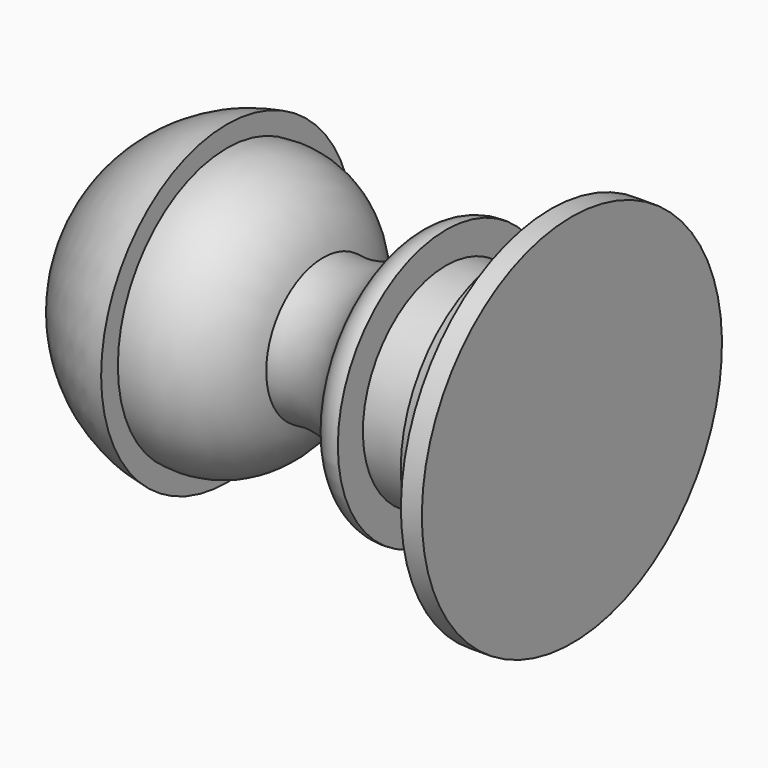
from build123d import *

# Parameters (mm, degrees)
F2_SCALE = 1.7


# Not quite as in the source:
# - a feature names something its author has since deleted; it is built from what else it names


with BuildPart() as f1:
    # F0 (on Front) → F1 (revolve)
    with BuildSketch(Plane.XZ):
        with BuildLine():
            Line((-7.3886374691, 0.0288757618), (0, 0.0425738979))
            Line((0, 0.0425738979), (0, 9))
            Line((0, 9), (-1, 9))
            ThreePointArc((-1, 9), (-1.5826778103, 7.4161422482), (-3, 6.5))
            Line((-3, 6.5), (-3, 5))
            Line((-3, 5), (-6, 5))
            Line((-6, 5), (-6, 6.5))
            ThreePointArc((-6, 6.5), (-6.9250133416, 6.2625200124), (-7.5, 5.5))
            Line((-7.5, 5.5), (-7.5, 0.0286693017))
            Line((-7.5, 0.0286693017), (-7.3886374691, 0.0288757618))
        make_face()
        with BuildLine():
            Line((-15.3639473664, 0.0140899666), (-7.5, 0.0286693017))
            Line((-7.5, 0.0286693017), (-7.5, 5.5))
            ThreePointArc((-7.5, 5.5), (-9.3734949345, 3.8129508491), (-11.8646939118, 3.4255934394))
            ThreePointArc((-11.8646939118, 3.4255934394), (-13.5762184414, 5.8486067414), (-16.4624222987, 6.534272091))
            Line((-16.4624222987, 6.534272091), (-16.4624222987, 7.534272091))
            ThreePointArc((-16.4624222987, 7.534272091), (-21.1178263748, 4.9792420326), (-22.9639343054, 0))
            Line((-22.9639343054, 0), (-15.3639473664, 0.0140899666))
        make_face()
    revolve(axis=Axis((-11.4639343054, 0, 0.0213203809), (0.9999982814, 0, 0.001853943)))


with BuildPart() as f2_1:
    # F2: copy of F1
    add(f1.part.scale(F2_SCALE))


solid = f2_1.part
